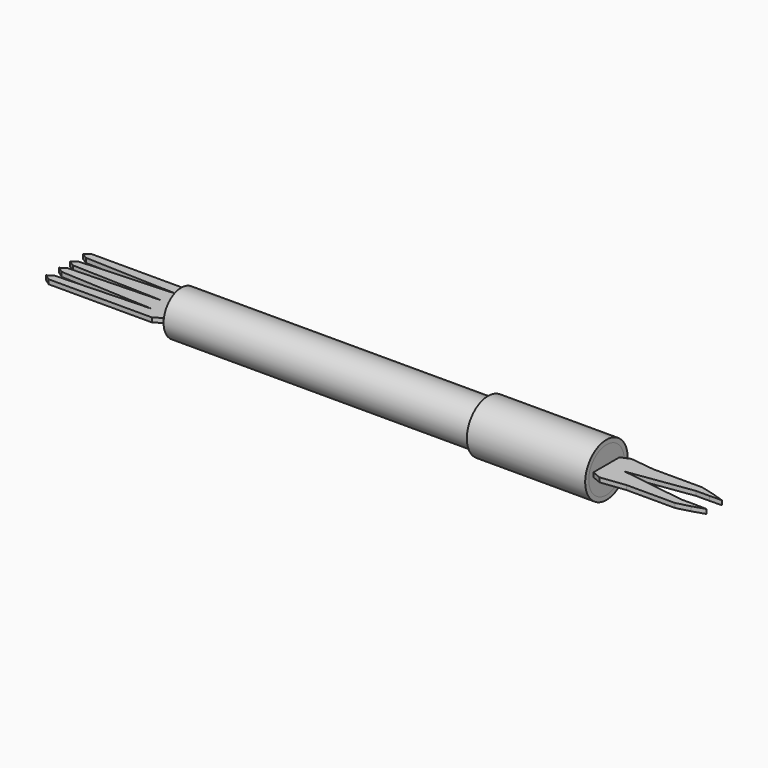
from build123d import *

# Parameters (mm, degrees)
F0_R     = 7.9375
F1_DEPTH = 152.4
F3_DEPTH = 1.5875
F5_DEPTH = 1.5875
F6_R     = 9.525
F6_R_2   = 7.9375
F7_DEPTH = 42.418


# Not quite as in the source:
# - a length typed as a fraction of an inch, garbled in the dataset ("3 / 203.2 mm" for 3/8 in), is restored
# - a feature names something its author has since deleted; it is built from what else it names


with BuildPart() as f1:
    # F0 (on Right) → F1 (new body)
    with BuildSketch(Plane.YZ):
        Circle(F0_R)
    extrude(amount=F1_DEPTH)

    # F4 (on Top) → F5 (join)
    with BuildSketch(Plane.XY):
        Polygon((155.6199789047, 7.1569969878), (152.3619145155, 5.799469538), (152.3619145155, 0), (159.0015292168, 0), (181.8202883005, 3.309753025), (186.6287142038, 3.309753025), (191.0549998283, 3.4116455354), (186.6287142038, 4.8380969092), (181.8202883005, 6.0837985948), (164.4826829433, 6.0837985948), align=None)
        Polygon((159.0015292168, 0), (152.3619145155, 0), (152.3619145155, -5.799469538), (155.6199789047, -7.1569969878), (164.4826829433, -6.0837985948), (181.8202883005, -6.0837985948), (186.6287142038, -4.8380969092), (191.0549998283, -3.4116455354), (186.6287142038, -3.309753025), (181.8202883005, -3.309753025), align=None)
    extrude(amount=F5_DEPTH)


with BuildPart() as f3:
    # F2 (on Top) → F3 (new body)
    with BuildSketch(Plane.XY):
        Polygon((0, 0), (0, 7.9797012731), (-2.7672210486, 9.7242689653), (-39.7654250264, 9.7242689653), (-41.8596901, 8.250253275), (-39.7654250264, 6.9576832621), (-5.9918332845, 5.6780572049), (-39.7654250264, 3.907465376), (-41.8596901, 2.4189068936), (-39.7654250264, 1.1263368807), (-6.7428140901, 0), align=None)
        Polygon((0, -7.9797012731), (0, 0), (-6.7428140901, 0), (-39.7654250264, -1.1263368807), (-41.8596901, -2.4189068936), (-39.7654250264, -3.907465376), (-5.9918332845, -5.6780572049), (-39.7654250264, -6.9576832621), (-41.8596901, -8.250253275), (-39.7654250264, -9.7242689653), (-2.7672210486, -9.7242689653), align=None)
    extrude(amount=F3_DEPTH)


with BuildPart() as f7:
    # F6 (on face) → F7 (new body)
    with BuildSketch(Plane.YZ.offset(152.4)):
        Circle(F6_R)
        Circle(F6_R_2, mode=Mode.SUBTRACT)
    extrude(amount=-F7_DEPTH)


solid = Compound([f1.part, f3.part, f7.part])
